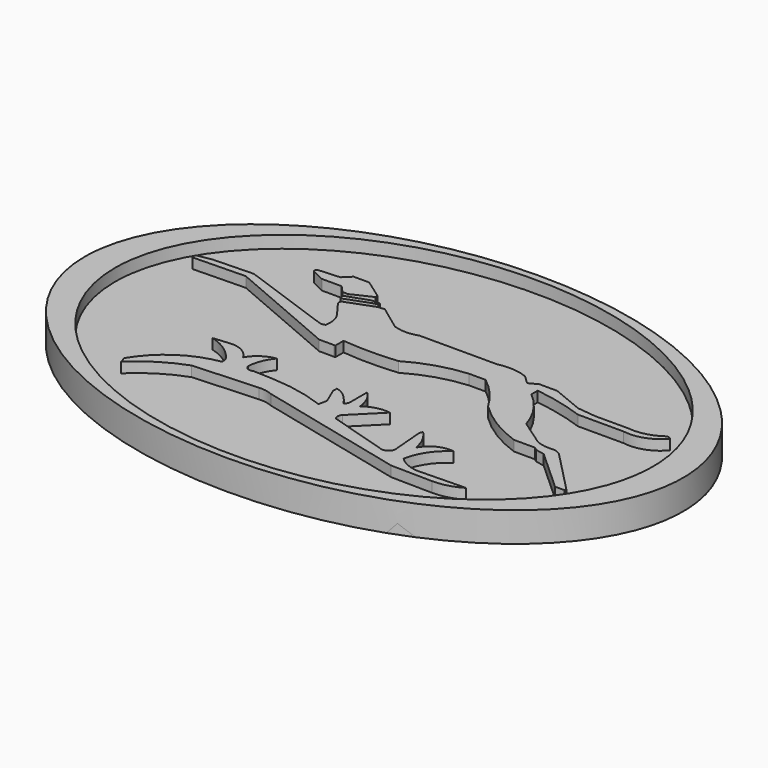
from build123d import *

# Parameters (mm, degrees)
F1_DEPTH = 5.588
F2_DEPTH = 9.525
F3_DEPTH = 8.89


with BuildPart() as f1:
    # F0 (on Top) → F1 (new body)
    with BuildSketch(Plane.XY):
        with BuildLine():
            add(Edge.make_bspline(
                [(-96.1296856403, 14.1812777147), (-96.1296856403, -95.1418774348), (48.0648428202, -40.4802998601), (192.2593712807, 14.1812777147), (48.0648428202, 68.8428552894), (-96.1296856403, 123.5044328642), (-96.1296856403, 14.1812777147)],
                knots=[0, 0, 0, 2.0943951024, 2.0943951024, 4.1887902048, 4.1887902048, 6.2831853072, 6.2831853072, 6.2831853072], degree=2, weights=[1, 0.5, 1, 0.5, 1, 0.5, 1]))
        make_face()
        with BuildLine():
            add(Edge.make_bspline(
                [(-86.4062830806, 14.1812777147), (-86.4062830806, -91.2685697716), (43.2031415403, -38.5436460285), (172.8125661612, 14.1812777147), (43.2031415403, 66.9062014578), (-86.4062830806, 119.631125201), (-86.4062830806, 14.1812777147)],
                knots=[0, 0, 0, 2.0943951024, 2.0943951024, 4.1887902048, 4.1887902048, 6.2831853072, 6.2831853072, 6.2831853072], degree=2, weights=[1, 0.5, 1, 0.5, 1, 0.5, 1]))
        make_face(mode=Mode.SUBTRACT)
        with BuildLine():
            add(Edge.make_bspline(
                [(-86.4062830806, 14.1812777147), (-86.4062830806, -91.2685697716), (43.2031415403, -38.5436460285), (172.8125661612, 14.1812777147), (43.2031415403, 66.9062014578), (-86.4062830806, 119.631125201), (-86.4062830806, 14.1812777147)],
                knots=[0, 0, 0, 2.0943951024, 2.0943951024, 4.1887902048, 4.1887902048, 6.2831853072, 6.2831853072, 6.2831853072], degree=2, weights=[1, 0.5, 1, 0.5, 1, 0.5, 1]))
        make_face()
        with BuildLine():
            ThreePointArc((-13.8349626213, -13.9056285843), (-15.9967648634, -13.2647105139), (-18.2475615293, -13.1302513182))
            Line((-18.2475615293, -13.1302513182), (-38.9931462705, -14.2642538995))
            ThreePointArc((-38.9931462705, -14.2642538995), (-47.064067943, -18.1789797213), (-54.1321523488, -23.7022973597))
            Line((-54.1321523488, -23.7022973597), (-54.7242574394, -21.6821748763))
            ThreePointArc((-54.7242574394, -21.6821748763), (-46.0878692508, -12.5354954755), (-34.3837179244, -7.9244449735))
            ThreePointArc((-34.3837179244, -7.9244449735), (-34.4701852634, -6.5814264399), (-35.0803136826, -5.3818770684))
            ThreePointArc((-35.0803136826, -5.3818770684), (-39.1636540714, -1.6431587661), (-44.2056916654, 0.6436600233))
            Line((-44.2056916654, 0.6436600233), (-39.0160679817, 1.131276018))
            ThreePointArc((-39.0160679817, 1.131276018), (-34.7883403032, 0.2781080389), (-31.7366607487, -2.7696499601))
            ThreePointArc((-31.7366607487, -2.7696499601), (-28.7662928335, 0.4349112266), (-24.7010625899, 2.0368478727))
            ThreePointArc((-24.7010625899, 2.0368478727), (-26.8360381128, -1.5534309837), (-27.7660768479, -5.6256847456))
            ThreePointArc((-27.7660768479, -5.6256847456), (-26.7479831914, -6.9858867275), (-25.049360469, -6.9492128678))
            Line((-25.049360469, -6.9492128678), (-18.4665471315, -7.2278501466))
            ThreePointArc((-18.4665471315, -7.2278501466), (-9.6347298239, -8.3104134806), (-1.0865301592, -10.7804788277))
            Line((-1.0865301592, -10.7804788277), (-0.4944257089, -8.0985920504))
            Line((-0.4944257089, -8.0985920504), (-2.7235259768, -2.8741385322))
            Line((-2.7235259768, -2.8741385322), (-2.7235259768, -1.3416317524))
            Line((-2.7235259768, -1.3416317524), (-1.0865301592, -1.8292476889))
            ThreePointArc((-1.0865301592, -1.8292476889), (1.5242180961, -3.9291084152), (3.5458186176, -6.6009154543))
            Line((3.5458186176, -6.6009154543), (4.4862208888, -5.6953430176))
            Line((4.4862208888, -5.6953430176), (4.4862208888, 1.827870612))
            ThreePointArc((4.4862208888, 1.827870612), (6.8143845426, -1.3780052873), (7.8298710287, -5.2077276632))
            ThreePointArc((7.8298710287, -5.2077276632), (11.6145293863, -3.3948152664), (15.8058721572, -3.1876051798))
            Line((15.8058721572, -3.1876051798), (7.3422566056, -11.6512207314))
            ThreePointArc((7.3422566056, -11.6512207314), (6.8084600077, -12.9399197176), (7.3422566056, -14.2286187038))
            Line((7.3422566056, -14.2286187038), (26.3244397938, -19.9755188078))
            ThreePointArc((26.3244397938, -19.9755188078), (28.6267380344, -19.4275469464), (29.2849633843, -17.1543136239))
            Line((29.2849633843, -17.1543136239), (28.4490510821, -7.2278473526))
            Line((28.4490510821, -7.2278473526), (28.9018359035, -6.2177861109))
            ThreePointArc((28.9018359035, -6.2177861109), (31.4390104817, -9.7818190159), (32.767932862, -13.9499781653))
            ThreePointArc((32.767932862, -13.9499781653), (36.4087946947, -10.4279306935), (41.4056964219, -9.5962658525))
            ThreePointArc((41.4056964219, -9.5962658525), (36.6190242076, -14.3289066551), (34.0914614499, -20.5676201731))
            ThreePointArc((34.0914614499, -20.5676201731), (37.1515055768, -22.656488899), (40.743932128, -23.5629733652))
            Line((40.743932128, -23.5629733652), (56.27797544, -23.2146773487))
            ThreePointArc((56.27797544, -23.2146773487), (51.9217919189, -25.0713695391), (47.2222566605, -25.6527550519))
            Line((47.2222566605, -25.6527550519), (33.9872011983, -25.4300821549))
            Line((33.9872011983, -25.4300821549), (-13.8349626213, -13.9056285843))
        make_face(mode=Mode.SUBTRACT)
        with BuildLine():
            Line((-39.7977419198, 46.4556999505), (-37.4409966171, 48.7782731652))
            Line((-37.4409966171, 48.7782731652), (-32.4272885919, 48.7782731652))
            Line((-32.4272885919, 48.7782731652), (-26.2392014265, 44.3969257176))
            Line((-26.2392014265, 44.3969257176), (-26.2392014265, 43.538723141))
            Line((-26.2392014265, 43.538723141), (-32.6079651713, 40.535017848))
            Line((-32.6079651713, 40.535017848), (-34.4147048891, 40.535017848))
            Line((-34.4147048891, 40.535017848), (-36.5602113307, 42.8611971438))
            Line((-36.5602113307, 42.8611971438), (-42.8838022053, 42.8611971438))
            Line((-42.8838022053, 42.8611971438), (-47.0618903637, 44.8711961508))
            ThreePointArc((-47.0618903637, 44.8711961508), (-47.1350933511, 45.603722533), (-46.5274862945, 46.0193753242))
            Line((-46.5274862945, 46.0193753242), (-39.7977419198, 46.4556999505))
        make_face(mode=Mode.SUBTRACT)
        with BuildLine():
            ThreePointArc((-31.9373272359, 37.7918481827), (-33.006023765, 38.091534076), (-32.6402410865, 39.1394495964))
            Line((-32.6402410865, 39.1394495964), (-25.8453879505, 41.527044028))
            Line((-25.8453879505, 41.527044028), (-23.1215879321, 41.527044028))
            Line((-23.1215879321, 41.527044028), (-23.1215879321, 40.7946519554))
            Line((-23.1215879321, 40.7946519554), (-24.6152840555, 40.5456386507))
            Line((-24.6152840555, 40.5456386507), (-31.9373272359, 37.7918481827))
        make_face(mode=Mode.SUBTRACT)
        with BuildLine():
            Line((-31.4023745043, 36.3093186869), (-22.3413072526, 39.7171489894))
            Line((-22.3413072526, 39.7171489894), (-20.2442985028, 39.851911366))
            Line((-20.2442985028, 39.851911366), (-12.4154109508, 34.0977273881))
            ThreePointArc((-12.4154109508, 34.0977273881), (-8.4577132948, 33.4132000605), (-4.5000156388, 34.0977273881))
            Line((-4.5000156388, 34.0977273881), (20.4140171409, 34.0977273881))
            ThreePointArc((20.4140171409, 34.0977273881), (25.2412459814, 34.4816780729), (29.9570616335, 33.3813875914))
            Line((29.9570616335, 33.3813875914), (32.4792265892, 30.9828575701))
            Line((32.4792265892, 30.9828575701), (33.1382118165, 30.9828575701))
            Line((33.1382118165, 30.9828575701), (33.7140932679, 31.2817543745))
            Line((33.7140932679, 31.2817543745), (35.176936537, 32.2593674064))
            Line((35.176936537, 32.2593674064), (41.1630272865, 32.2593674064))
            Line((41.1630272865, 32.2593674064), (51.1939786375, 28.1484182924))
            Line((51.1939786375, 28.1484182924), (57.1150295436, 27.4817384779))
            Line((57.1150295436, 27.4817384779), (67.8917467594, 27.4817384779))
            ThreePointArc((67.8917467594, 27.4817384779), (73.2037929102, 27.8324149258), (78.0254527926, 30.0890505314))
            ThreePointArc((78.0254527926, 30.0890505314), (78.8384481256, 30.0565583066), (79.5194506645, 29.6113025397))
            ThreePointArc((79.5194506645, 29.6113025397), (74.2653604379, 26.0014945743), (67.9170712829, 25.4223551601))
            Line((67.9170712829, 25.4223551601), (53.3066615462, 25.4223551601))
            ThreePointArc((53.3066615462, 25.4223551601), (45.4053992725, 27.7792179463), (37.299670279, 29.2898155749))
            Line((37.299670279, 29.2898155749), (37.299670279, 26.7115086317))
            ThreePointArc((37.299670279, 26.7115086317), (42.7871554302, 20.7116696997), (46.3237427175, 13.3902551606))
            Line((46.3237427175, 13.3902551606), (54.649528116, 7.6427781023))
            ThreePointArc((54.649528116, 7.6427781023), (57.0349413033, 6.8724866612), (59.5375671983, 6.7296279594))
            ThreePointArc((59.5375671983, 6.7296279594), (61.5128703178, 6.5524358643), (63.1901696324, 5.494188983))
            Line((63.1901696324, 5.494188983), (76.2965604663, -7.9882089049))
            Line((76.2965604663, -7.9882089049), (76.2965604663, -8.7402155623))
            Line((76.2965604663, -8.7402155623), (73.2885375619, -8.7402155623))
            Line((73.2885375619, -8.7402155623), (59.9672868848, 3.3455996308))
            Line((59.9672868848, 3.3455996308), (57.0129752159, 3.9364616387))
            Line((57.0129752159, 3.9364616387), (56.0998246074, 4.6884673648))
            Line((56.0998246074, 4.6884673648), (49.3317693472, 4.6884673648))
            ThreePointArc((49.3317693472, 4.6884673648), (40.5518576369, 8.8563602175), (32.8950583935, 14.8423109204))
            ThreePointArc((32.8950583935, 14.8423109204), (28.6936482169, 20.7266141239), (23.4412644058, 25.695450604))
            Line((23.4412644058, 25.695450604), (18.0697888136, 25.695450604))
            ThreePointArc((18.0697888136, 25.695450604), (8.7134500786, 23.8677238781), (0, 20.0002379715))
            ThreePointArc((0, 20.0002379715), (-8.8261405876, 19.5700583027), (-17.6522811752, 20.0002379715))
            Line((-17.6522811752, 20.0002379715), (-17.6522811752, 16.719225047))
            Line((-17.6522811752, 16.719225047), (-18.1164946407, 16.7051069438))
            Line((-18.1164946407, 16.7051069438), (-22.8311270475, 16.7051069438))
            Line((-22.8311270475, 16.7051069438), (-58.7315559387, 32.1072898805))
            Line((-58.7315559387, 32.1072898805), (-75.6004303694, 31.7179113626))
            ThreePointArc((-75.6004303694, 31.7179113626), (-75.7728203102, 32.4162039785), (-75.557179749, 33.1023745239))
            Line((-75.557179749, 33.1023745239), (-70.7560405135, 33.967666328))
            Line((-70.7560405135, 33.967666328), (-57.9529926181, 34.3570448458))
            Line((-57.9529926181, 34.3570448458), (-28.6270994693, 23.8870233297))
            ThreePointArc((-28.6270994693, 23.8870233297), (-27.5911867091, 23.7266136467), (-26.5693385154, 23.960435763))
            ThreePointArc((-26.5693385154, 23.960435763), (-26.568177582, 27.2335095867), (-27.9155671597, 30.2163865417))
            Line((-27.9155671597, 30.2163865417), (-31.4023745043, 34.9330492318))
            ThreePointArc((-31.4023745043, 34.9330492318), (-31.6025112053, 35.6211839593), (-31.4023745043, 36.3093186869))
        make_face(mode=Mode.SUBTRACT)
        with BuildLine():
            Line((-32.4272885919, 48.7782731652), (-37.4409966171, 48.7782731652))
            Line((-37.4409966171, 48.7782731652), (-39.7977419198, 46.4556999505))
            Line((-39.7977419198, 46.4556999505), (-46.5274862945, 46.0193753242))
            ThreePointArc((-46.5274862945, 46.0193753242), (-47.1350933511, 45.603722533), (-47.0618903637, 44.8711961508))
            Line((-47.0618903637, 44.8711961508), (-42.8838022053, 42.8611971438))
            Line((-42.8838022053, 42.8611971438), (-36.5602113307, 42.8611971438))
            Line((-36.5602113307, 42.8611971438), (-34.4147048891, 40.535017848))
            Line((-34.4147048891, 40.535017848), (-32.6079651713, 40.535017848))
            Line((-32.6079651713, 40.535017848), (-26.2392014265, 43.538723141))
            Line((-26.2392014265, 43.538723141), (-26.2392014265, 44.3969257176))
            Line((-26.2392014265, 44.3969257176), (-32.4272885919, 48.7782731652))
        make_face()
        with BuildLine():
            Line((-25.8453879505, 41.527044028), (-32.6402410865, 39.1394495964))
            ThreePointArc((-32.6402410865, 39.1394495964), (-33.006023765, 38.091534076), (-31.9373272359, 37.7918481827))
            Line((-31.9373272359, 37.7918481827), (-24.6152840555, 40.5456386507))
            Line((-24.6152840555, 40.5456386507), (-23.1215879321, 40.7946519554))
            Line((-23.1215879321, 40.7946519554), (-23.1215879321, 41.527044028))
            Line((-23.1215879321, 41.527044028), (-25.8453879505, 41.527044028))
        make_face()
        with BuildLine():
            Line((-20.2442985028, 39.851911366), (-22.3413072526, 39.7171489894))
            Line((-22.3413072526, 39.7171489894), (-31.4023745043, 36.3093186869))
            ThreePointArc((-31.4023745043, 36.3093186869), (-31.6025112053, 35.6211839593), (-31.4023745043, 34.9330492318))
            Line((-31.4023745043, 34.9330492318), (-27.9155671597, 30.2163865417))
            ThreePointArc((-27.9155671597, 30.2163865417), (-26.568177582, 27.2335095867), (-26.5693385154, 23.960435763))
            ThreePointArc((-26.5693385154, 23.960435763), (-27.5911867091, 23.7266136467), (-28.6270994693, 23.8870233297))
            Line((-28.6270994693, 23.8870233297), (-57.9529926181, 34.3570448458))
            Line((-57.9529926181, 34.3570448458), (-70.7560405135, 33.967666328))
            Line((-70.7560405135, 33.967666328), (-75.557179749, 33.1023745239))
            ThreePointArc((-75.557179749, 33.1023745239), (-75.7728203102, 32.4162039785), (-75.6004303694, 31.7179113626))
            Line((-75.6004303694, 31.7179113626), (-58.7315559387, 32.1072898805))
            Line((-58.7315559387, 32.1072898805), (-22.8311270475, 16.7051069438))
            Line((-22.8311270475, 16.7051069438), (-18.1164946407, 16.7051069438))
            Line((-18.1164946407, 16.7051069438), (-17.6522811752, 16.719225047))
            Line((-17.6522811752, 16.719225047), (-17.6522811752, 20.0002379715))
            ThreePointArc((-17.6522811752, 20.0002379715), (-8.8261405876, 19.5700583027), (0, 20.0002379715))
            ThreePointArc((0, 20.0002379715), (8.7134500786, 23.8677238781), (18.0697888136, 25.695450604))
            Line((18.0697888136, 25.695450604), (23.4412644058, 25.695450604))
            ThreePointArc((23.4412644058, 25.695450604), (28.6936482169, 20.7266141239), (32.8950583935, 14.8423109204))
            ThreePointArc((32.8950583935, 14.8423109204), (40.5518576369, 8.8563602175), (49.3317693472, 4.6884673648))
            Line((49.3317693472, 4.6884673648), (56.0998246074, 4.6884673648))
            Line((56.0998246074, 4.6884673648), (57.0129752159, 3.9364616387))
            Line((57.0129752159, 3.9364616387), (59.9672868848, 3.3455996308))
            Line((59.9672868848, 3.3455996308), (73.2885375619, -8.7402155623))
            Line((73.2885375619, -8.7402155623), (76.2965604663, -8.7402155623))
            Line((76.2965604663, -8.7402155623), (76.2965604663, -7.9882089049))
            Line((76.2965604663, -7.9882089049), (63.1901696324, 5.494188983))
            ThreePointArc((63.1901696324, 5.494188983), (61.5128703178, 6.5524358643), (59.5375671983, 6.7296279594))
            ThreePointArc((59.5375671983, 6.7296279594), (57.0349413033, 6.8724866612), (54.649528116, 7.6427781023))
            Line((54.649528116, 7.6427781023), (46.3237427175, 13.3902551606))
            ThreePointArc((46.3237427175, 13.3902551606), (42.7871554302, 20.7116696997), (37.299670279, 26.7115086317))
            Line((37.299670279, 26.7115086317), (37.299670279, 29.2898155749))
            ThreePointArc((37.299670279, 29.2898155749), (45.4053992725, 27.7792179463), (53.3066615462, 25.4223551601))
            Line((53.3066615462, 25.4223551601), (67.9170712829, 25.4223551601))
            ThreePointArc((67.9170712829, 25.4223551601), (74.2653604379, 26.0014945743), (79.5194506645, 29.6113025397))
            ThreePointArc((79.5194506645, 29.6113025397), (78.8384481256, 30.0565583066), (78.0254527926, 30.0890505314))
            ThreePointArc((78.0254527926, 30.0890505314), (73.2037929102, 27.8324149258), (67.8917467594, 27.4817384779))
            Line((67.8917467594, 27.4817384779), (57.1150295436, 27.4817384779))
            Line((57.1150295436, 27.4817384779), (51.1939786375, 28.1484182924))
            Line((51.1939786375, 28.1484182924), (41.1630272865, 32.2593674064))
            Line((41.1630272865, 32.2593674064), (35.176936537, 32.2593674064))
            Line((35.176936537, 32.2593674064), (33.7140932679, 31.2817543745))
            Line((33.7140932679, 31.2817543745), (33.1382118165, 30.9828575701))
            Line((33.1382118165, 30.9828575701), (32.4792265892, 30.9828575701))
            Line((32.4792265892, 30.9828575701), (29.9570616335, 33.3813875914))
            ThreePointArc((29.9570616335, 33.3813875914), (25.2412459814, 34.4816780729), (20.4140171409, 34.0977273881))
            Line((20.4140171409, 34.0977273881), (-4.5000156388, 34.0977273881))
            ThreePointArc((-4.5000156388, 34.0977273881), (-8.4577132948, 33.4132000605), (-12.4154109508, 34.0977273881))
            Line((-12.4154109508, 34.0977273881), (-20.2442985028, 39.851911366))
        make_face()
        with BuildLine():
            Line((-38.9931462705, -14.2642538995), (-18.2475615293, -13.1302513182))
            ThreePointArc((-18.2475615293, -13.1302513182), (-15.9967648634, -13.2647105139), (-13.8349626213, -13.9056285843))
            Line((-13.8349626213, -13.9056285843), (33.9872011983, -25.4300821549))
            Line((33.9872011983, -25.4300821549), (47.2222566605, -25.6527550519))
            ThreePointArc((47.2222566605, -25.6527550519), (51.9217919189, -25.0713695391), (56.27797544, -23.2146773487))
            Line((56.27797544, -23.2146773487), (40.743932128, -23.5629733652))
            ThreePointArc((40.743932128, -23.5629733652), (37.1515055768, -22.656488899), (34.0914614499, -20.5676201731))
            ThreePointArc((34.0914614499, -20.5676201731), (36.6190242076, -14.3289066551), (41.4056964219, -9.5962658525))
            ThreePointArc((41.4056964219, -9.5962658525), (36.4087946947, -10.4279306935), (32.767932862, -13.9499781653))
            ThreePointArc((32.767932862, -13.9499781653), (31.4390104817, -9.7818190159), (28.9018359035, -6.2177861109))
            Line((28.9018359035, -6.2177861109), (28.4490510821, -7.2278473526))
            Line((28.4490510821, -7.2278473526), (29.2849633843, -17.1543136239))
            ThreePointArc((29.2849633843, -17.1543136239), (28.6267380344, -19.4275469464), (26.3244397938, -19.9755188078))
            Line((26.3244397938, -19.9755188078), (7.3422566056, -14.2286187038))
            ThreePointArc((7.3422566056, -14.2286187038), (6.8084600077, -12.9399197176), (7.3422566056, -11.6512207314))
            Line((7.3422566056, -11.6512207314), (15.8058721572, -3.1876051798))
            ThreePointArc((15.8058721572, -3.1876051798), (11.6145293863, -3.3948152664), (7.8298710287, -5.2077276632))
            ThreePointArc((7.8298710287, -5.2077276632), (6.8143845426, -1.3780052873), (4.4862208888, 1.827870612))
            Line((4.4862208888, 1.827870612), (4.4862208888, -5.6953430176))
            Line((4.4862208888, -5.6953430176), (3.5458186176, -6.6009154543))
            ThreePointArc((3.5458186176, -6.6009154543), (1.5242180961, -3.9291084152), (-1.0865301592, -1.8292476889))
            Line((-1.0865301592, -1.8292476889), (-2.7235259768, -1.3416317524))
            Line((-2.7235259768, -1.3416317524), (-2.7235259768, -2.8741385322))
            Line((-2.7235259768, -2.8741385322), (-0.4944257089, -8.0985920504))
            Line((-0.4944257089, -8.0985920504), (-1.0865301592, -10.7804788277))
            ThreePointArc((-1.0865301592, -10.7804788277), (-9.6347298239, -8.3104134806), (-18.4665471315, -7.2278501466))
            Line((-18.4665471315, -7.2278501466), (-25.049360469, -6.9492128678))
            ThreePointArc((-25.049360469, -6.9492128678), (-26.7479831914, -6.9858867275), (-27.7660768479, -5.6256847456))
            ThreePointArc((-27.7660768479, -5.6256847456), (-26.8360381128, -1.5534309837), (-24.7010625899, 2.0368478727))
            ThreePointArc((-24.7010625899, 2.0368478727), (-28.7662928335, 0.4349112266), (-31.7366607487, -2.7696499601))
            ThreePointArc((-31.7366607487, -2.7696499601), (-34.7883403032, 0.2781080389), (-39.0160679817, 1.131276018))
            Line((-39.0160679817, 1.131276018), (-44.2056916654, 0.6436600233))
            ThreePointArc((-44.2056916654, 0.6436600233), (-39.1636540714, -1.6431587661), (-35.0803136826, -5.3818770684))
            ThreePointArc((-35.0803136826, -5.3818770684), (-34.4701852634, -6.5814264399), (-34.3837179244, -7.9244449735))
            ThreePointArc((-34.3837179244, -7.9244449735), (-46.0878692508, -12.5354954755), (-54.7242574394, -21.6821748763))
            Line((-54.7242574394, -21.6821748763), (-54.1321523488, -23.7022973597))
            ThreePointArc((-54.1321523488, -23.7022973597), (-47.064067943, -18.1789797213), (-38.9931462705, -14.2642538995))
        make_face()
    extrude(amount=F1_DEPTH)


with BuildPart() as f2:
    # F0 (on Top) → F2 (new body)
    with BuildSketch(Plane.XY):
        with BuildLine():
            add(Edge.make_bspline(
                [(-96.1296856403, 14.1812777147), (-96.1296856403, -95.1418774348), (48.0648428202, -40.4802998601), (192.2593712807, 14.1812777147), (48.0648428202, 68.8428552894), (-96.1296856403, 123.5044328642), (-96.1296856403, 14.1812777147)],
                knots=[0, 0, 0, 2.0943951024, 2.0943951024, 4.1887902048, 4.1887902048, 6.2831853072, 6.2831853072, 6.2831853072], degree=2, weights=[1, 0.5, 1, 0.5, 1, 0.5, 1]))
        make_face()
        with BuildLine():
            add(Edge.make_bspline(
                [(-86.4062830806, 14.1812777147), (-86.4062830806, -91.2685697716), (43.2031415403, -38.5436460285), (172.8125661612, 14.1812777147), (43.2031415403, 66.9062014578), (-86.4062830806, 119.631125201), (-86.4062830806, 14.1812777147)],
                knots=[0, 0, 0, 2.0943951024, 2.0943951024, 4.1887902048, 4.1887902048, 6.2831853072, 6.2831853072, 6.2831853072], degree=2, weights=[1, 0.5, 1, 0.5, 1, 0.5, 1]))
        make_face(mode=Mode.SUBTRACT)
    extrude(amount=F2_DEPTH)


with BuildPart() as f3:
    # F0 (on Top) → F3 (new body)
    with BuildSketch(Plane.XY):
        with BuildLine():
            Line((-32.4272885919, 48.7782731652), (-37.4409966171, 48.7782731652))
            Line((-37.4409966171, 48.7782731652), (-39.7977419198, 46.4556999505))
            Line((-39.7977419198, 46.4556999505), (-46.5274862945, 46.0193753242))
            ThreePointArc((-46.5274862945, 46.0193753242), (-47.1350933511, 45.603722533), (-47.0618903637, 44.8711961508))
            Line((-47.0618903637, 44.8711961508), (-42.8838022053, 42.8611971438))
            Line((-42.8838022053, 42.8611971438), (-36.5602113307, 42.8611971438))
            Line((-36.5602113307, 42.8611971438), (-34.4147048891, 40.535017848))
            Line((-34.4147048891, 40.535017848), (-32.6079651713, 40.535017848))
            Line((-32.6079651713, 40.535017848), (-26.2392014265, 43.538723141))
            Line((-26.2392014265, 43.538723141), (-26.2392014265, 44.3969257176))
            Line((-26.2392014265, 44.3969257176), (-32.4272885919, 48.7782731652))
        make_face()
    extrude(amount=F3_DEPTH)


with BuildPart() as f3b:
    # F0 (on Top) → F3, piece 2 (new body)
    with BuildSketch(Plane.XY):
        with BuildLine():
            Line((-25.8453879505, 41.527044028), (-32.6402410865, 39.1394495964))
            ThreePointArc((-32.6402410865, 39.1394495964), (-33.006023765, 38.091534076), (-31.9373272359, 37.7918481827))
            Line((-31.9373272359, 37.7918481827), (-24.6152840555, 40.5456386507))
            Line((-24.6152840555, 40.5456386507), (-23.1215879321, 40.7946519554))
            Line((-23.1215879321, 40.7946519554), (-23.1215879321, 41.527044028))
            Line((-23.1215879321, 41.527044028), (-25.8453879505, 41.527044028))
        make_face()
    extrude(amount=F3_DEPTH)


with BuildPart() as f3c:
    # F0 (on Top) → F3, piece 3 (new body)
    with BuildSketch(Plane.XY):
        with BuildLine():
            Line((-20.2442985028, 39.851911366), (-22.3413072526, 39.7171489894))
            Line((-22.3413072526, 39.7171489894), (-31.4023745043, 36.3093186869))
            ThreePointArc((-31.4023745043, 36.3093186869), (-31.6025112053, 35.6211839593), (-31.4023745043, 34.9330492318))
            Line((-31.4023745043, 34.9330492318), (-27.9155671597, 30.2163865417))
            ThreePointArc((-27.9155671597, 30.2163865417), (-26.568177582, 27.2335095867), (-26.5693385154, 23.960435763))
            ThreePointArc((-26.5693385154, 23.960435763), (-27.5911867091, 23.7266136467), (-28.6270994693, 23.8870233297))
            Line((-28.6270994693, 23.8870233297), (-57.9529926181, 34.3570448458))
            Line((-57.9529926181, 34.3570448458), (-70.7560405135, 33.967666328))
            Line((-70.7560405135, 33.967666328), (-75.557179749, 33.1023745239))
            ThreePointArc((-75.557179749, 33.1023745239), (-75.7728203102, 32.4162039785), (-75.6004303694, 31.7179113626))
            Line((-75.6004303694, 31.7179113626), (-58.7315559387, 32.1072898805))
            Line((-58.7315559387, 32.1072898805), (-22.8311270475, 16.7051069438))
            Line((-22.8311270475, 16.7051069438), (-18.1164946407, 16.7051069438))
            Line((-18.1164946407, 16.7051069438), (-17.6522811752, 16.719225047))
            Line((-17.6522811752, 16.719225047), (-17.6522811752, 20.0002379715))
            ThreePointArc((-17.6522811752, 20.0002379715), (-8.8261405876, 19.5700583027), (0, 20.0002379715))
            ThreePointArc((0, 20.0002379715), (8.7134500786, 23.8677238781), (18.0697888136, 25.695450604))
            Line((18.0697888136, 25.695450604), (23.4412644058, 25.695450604))
            ThreePointArc((23.4412644058, 25.695450604), (28.6936482169, 20.7266141239), (32.8950583935, 14.8423109204))
            ThreePointArc((32.8950583935, 14.8423109204), (40.5518576369, 8.8563602175), (49.3317693472, 4.6884673648))
            Line((49.3317693472, 4.6884673648), (56.0998246074, 4.6884673648))
            Line((56.0998246074, 4.6884673648), (57.0129752159, 3.9364616387))
            Line((57.0129752159, 3.9364616387), (59.9672868848, 3.3455996308))
            Line((59.9672868848, 3.3455996308), (73.2885375619, -8.7402155623))
            Line((73.2885375619, -8.7402155623), (76.2965604663, -8.7402155623))
            Line((76.2965604663, -8.7402155623), (76.2965604663, -7.9882089049))
            Line((76.2965604663, -7.9882089049), (63.1901696324, 5.494188983))
            ThreePointArc((63.1901696324, 5.494188983), (61.5128703178, 6.5524358643), (59.5375671983, 6.7296279594))
            ThreePointArc((59.5375671983, 6.7296279594), (57.0349413033, 6.8724866612), (54.649528116, 7.6427781023))
            Line((54.649528116, 7.6427781023), (46.3237427175, 13.3902551606))
            ThreePointArc((46.3237427175, 13.3902551606), (42.7871554302, 20.7116696997), (37.299670279, 26.7115086317))
            Line((37.299670279, 26.7115086317), (37.299670279, 29.2898155749))
            ThreePointArc((37.299670279, 29.2898155749), (45.4053992725, 27.7792179463), (53.3066615462, 25.4223551601))
            Line((53.3066615462, 25.4223551601), (67.9170712829, 25.4223551601))
            ThreePointArc((67.9170712829, 25.4223551601), (74.2653604379, 26.0014945743), (79.5194506645, 29.6113025397))
            ThreePointArc((79.5194506645, 29.6113025397), (78.8384481256, 30.0565583066), (78.0254527926, 30.0890505314))
            ThreePointArc((78.0254527926, 30.0890505314), (73.2037929102, 27.8324149258), (67.8917467594, 27.4817384779))
            Line((67.8917467594, 27.4817384779), (57.1150295436, 27.4817384779))
            Line((57.1150295436, 27.4817384779), (51.1939786375, 28.1484182924))
            Line((51.1939786375, 28.1484182924), (41.1630272865, 32.2593674064))
            Line((41.1630272865, 32.2593674064), (35.176936537, 32.2593674064))
            Line((35.176936537, 32.2593674064), (33.7140932679, 31.2817543745))
            Line((33.7140932679, 31.2817543745), (33.1382118165, 30.9828575701))
            Line((33.1382118165, 30.9828575701), (32.4792265892, 30.9828575701))
            Line((32.4792265892, 30.9828575701), (29.9570616335, 33.3813875914))
            ThreePointArc((29.9570616335, 33.3813875914), (25.2412459814, 34.4816780729), (20.4140171409, 34.0977273881))
            Line((20.4140171409, 34.0977273881), (-4.5000156388, 34.0977273881))
            ThreePointArc((-4.5000156388, 34.0977273881), (-8.4577132948, 33.4132000605), (-12.4154109508, 34.0977273881))
            Line((-12.4154109508, 34.0977273881), (-20.2442985028, 39.851911366))
        make_face()
    extrude(amount=F3_DEPTH)


with BuildPart() as f3d:
    # F0 (on Top) → F3, piece 4 (new body)
    with BuildSketch(Plane.XY):
        with BuildLine():
            Line((-38.9931462705, -14.2642538995), (-18.2475615293, -13.1302513182))
            ThreePointArc((-18.2475615293, -13.1302513182), (-15.9967648634, -13.2647105139), (-13.8349626213, -13.9056285843))
            Line((-13.8349626213, -13.9056285843), (33.9872011983, -25.4300821549))
            Line((33.9872011983, -25.4300821549), (47.2222566605, -25.6527550519))
            ThreePointArc((47.2222566605, -25.6527550519), (51.9217919189, -25.0713695391), (56.27797544, -23.2146773487))
            Line((56.27797544, -23.2146773487), (40.743932128, -23.5629733652))
            ThreePointArc((40.743932128, -23.5629733652), (37.1515055768, -22.656488899), (34.0914614499, -20.5676201731))
            ThreePointArc((34.0914614499, -20.5676201731), (36.6190242076, -14.3289066551), (41.4056964219, -9.5962658525))
            ThreePointArc((41.4056964219, -9.5962658525), (36.4087946947, -10.4279306935), (32.767932862, -13.9499781653))
            ThreePointArc((32.767932862, -13.9499781653), (31.4390104817, -9.7818190159), (28.9018359035, -6.2177861109))
            Line((28.9018359035, -6.2177861109), (28.4490510821, -7.2278473526))
            Line((28.4490510821, -7.2278473526), (29.2849633843, -17.1543136239))
            ThreePointArc((29.2849633843, -17.1543136239), (28.6267380344, -19.4275469464), (26.3244397938, -19.9755188078))
            Line((26.3244397938, -19.9755188078), (7.3422566056, -14.2286187038))
            ThreePointArc((7.3422566056, -14.2286187038), (6.8084600077, -12.9399197176), (7.3422566056, -11.6512207314))
            Line((7.3422566056, -11.6512207314), (15.8058721572, -3.1876051798))
            ThreePointArc((15.8058721572, -3.1876051798), (11.6145293863, -3.3948152664), (7.8298710287, -5.2077276632))
            ThreePointArc((7.8298710287, -5.2077276632), (6.8143845426, -1.3780052873), (4.4862208888, 1.827870612))
            Line((4.4862208888, 1.827870612), (4.4862208888, -5.6953430176))
            Line((4.4862208888, -5.6953430176), (3.5458186176, -6.6009154543))
            ThreePointArc((3.5458186176, -6.6009154543), (1.5242180961, -3.9291084152), (-1.0865301592, -1.8292476889))
            Line((-1.0865301592, -1.8292476889), (-2.7235259768, -1.3416317524))
            Line((-2.7235259768, -1.3416317524), (-2.7235259768, -2.8741385322))
            Line((-2.7235259768, -2.8741385322), (-0.4944257089, -8.0985920504))
            Line((-0.4944257089, -8.0985920504), (-1.0865301592, -10.7804788277))
            ThreePointArc((-1.0865301592, -10.7804788277), (-9.6347298239, -8.3104134806), (-18.4665471315, -7.2278501466))
            Line((-18.4665471315, -7.2278501466), (-25.049360469, -6.9492128678))
            ThreePointArc((-25.049360469, -6.9492128678), (-26.7479831914, -6.9858867275), (-27.7660768479, -5.6256847456))
            ThreePointArc((-27.7660768479, -5.6256847456), (-26.8360381128, -1.5534309837), (-24.7010625899, 2.0368478727))
            ThreePointArc((-24.7010625899, 2.0368478727), (-28.7662928335, 0.4349112266), (-31.7366607487, -2.7696499601))
            ThreePointArc((-31.7366607487, -2.7696499601), (-34.7883403032, 0.2781080389), (-39.0160679817, 1.131276018))
            Line((-39.0160679817, 1.131276018), (-44.2056916654, 0.6436600233))
            ThreePointArc((-44.2056916654, 0.6436600233), (-39.1636540714, -1.6431587661), (-35.0803136826, -5.3818770684))
            ThreePointArc((-35.0803136826, -5.3818770684), (-34.4701852634, -6.5814264399), (-34.3837179244, -7.9244449735))
            ThreePointArc((-34.3837179244, -7.9244449735), (-46.0878692508, -12.5354954755), (-54.7242574394, -21.6821748763))
            Line((-54.7242574394, -21.6821748763), (-54.1321523488, -23.7022973597))
            ThreePointArc((-54.1321523488, -23.7022973597), (-47.064067943, -18.1789797213), (-38.9931462705, -14.2642538995))
        make_face()
    extrude(amount=F3_DEPTH)


solid = Compound([f1.part, f2.part, f3.part, f3b.part, f3c.part, f3d.part])
